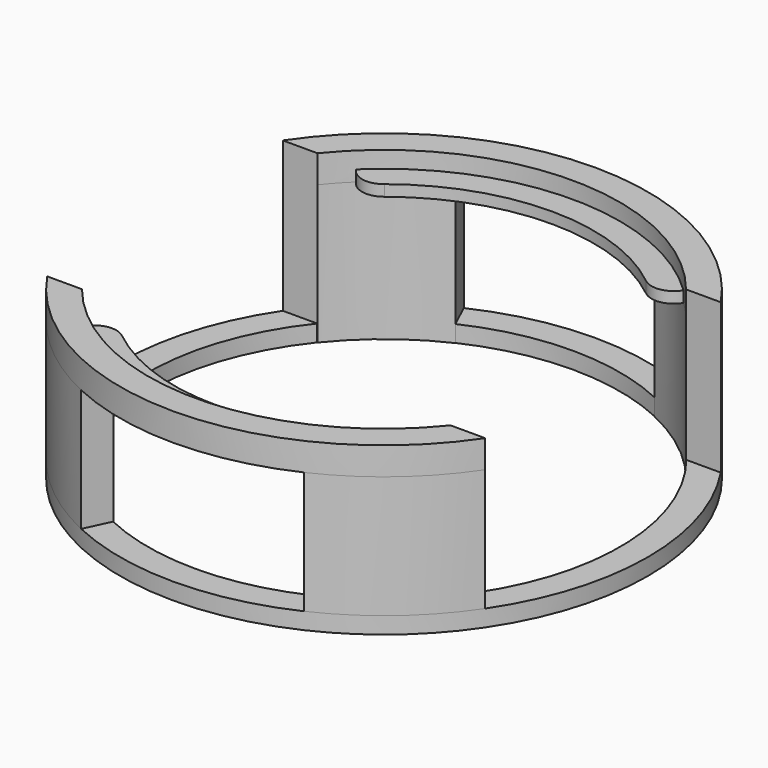
from build123d import *

# Parameters (mm, degrees)
F0_R        = 47.5
F0_R_2      = 42.5
F1_DEPTH    = 3
F3_DEPTH    = 25
F7_DEPTH    = 5
F8_DEPTH    = 2
F9_T1_DEPTH = 43.7405186698


# Not quite as in the source:
# - a fillet or chamfer that OpenCascade refuses, or shapes differently, is made with other operations: its cross-section is extruded or revolved along the edge and cut away or added


with BuildPart() as f1:
    # F0 (on Top) → F1 (new body)
    with BuildSketch(Plane.XY):
        Circle(F0_R)
        Circle(F0_R_2, mode=Mode.SUBTRACT)
    extrude(amount=F1_DEPTH)

    # F2 (on Top) → F3 (join)
    with BuildSketch(Plane.XY):
        with BuildLine():
            Line((-17.9424604553, 38.4777306174), (-20.0743674327, 43.0496198842))
            ThreePointArc((-20.0743674327, 43.0496198842), (-30.8770370262, 36.0951324209), (-39.4208066889, 26.5))
            Line((-39.4208066889, 26.5), (-33.1695287976, 26.5))
            ThreePointArc((-33.1695287976, 26.5), (-26.2483403101, 33.3690316255), (-17.9424604553, 38.4777306174))
        make_face()
        with BuildLine():
            Line((-20.0743674327, -43.0496198842), (-17.9424604553, -38.4777306174))
            ThreePointArc((-17.9424604553, -38.4777306174), (-26.2483403101, -33.3690316255), (-33.1695287976, -26.5))
            Line((-33.1695287976, -26.5), (-39.4208066889, -26.5))
            ThreePointArc((-39.4208066889, -26.5), (-30.8770370262, -36.0951324209), (-20.0743674327, -43.0496198842))
        make_face()
        with BuildLine():
            Line((20.0743674327, 43.0496198842), (17.9424604553, 38.4777306174))
            ThreePointArc((17.9424604553, 38.4777306174), (26.2483403101, 33.3690316255), (33.1695287976, 26.5))
            Line((33.1695287976, 26.5), (39.4208066889, 26.5))
            ThreePointArc((39.4208066889, 26.5), (30.8770370262, 36.0951324209), (20.0743674327, 43.0496198842))
        make_face()
        with BuildLine():
            ThreePointArc((33.1695287976, -26.5), (26.2483403101, -33.3690316255), (17.9424604553, -38.4777306174))
            Line((17.9424604553, -38.4777306174), (20.0743674327, -43.0496198842))
            ThreePointArc((20.0743674327, -43.0496198842), (30.8770370262, -36.0951324209), (39.4208066889, -26.5))
            Line((39.4208066889, -26.5), (33.1695287976, -26.5))
        make_face()
    extrude(amount=F3_DEPTH)

    # F4 (on face) → F7 (join)
    with BuildSketch(Plane.XY.offset(25)):
        with BuildLine():
            ThreePointArc((39.4208066889, 26.5), (0, 47.5), (-39.4208066889, 26.5))
            Line((-39.4208066889, 26.5), (-33.1695287976, 26.5))
            ThreePointArc((-33.1695287976, 26.5), (0, 42.455478335), (33.1695287976, 26.5))
            Line((33.1695287976, 26.5), (39.4208066889, 26.5))
        make_face()
        with BuildLine():
            Line((-33.1695287976, -26.5), (-39.4208066889, -26.5))
            ThreePointArc((-39.4208066889, -26.5), (0, -47.5), (39.4208066889, -26.5))
            Line((39.4208066889, -26.5), (33.1695287976, -26.5))
            ThreePointArc((33.1695287976, -26.5), (0, -42.455478335), (-33.1695287976, -26.5))
        make_face()
    extrude(amount=F7_DEPTH)

    # F6 (on offset) → F8 (join)
    with BuildSketch(Plane.XY.offset(25)):
        with BuildLine():
            ThreePointArc((-29.4712756106, -30.6217882215), (0, -42.5), (29.4712756106, -30.6217882215))
            Line((29.4712756106, -30.6217882215), (29.4712756106, -23.6217882215))
            ThreePointArc((29.4712756106, -23.6217882215), (0, -37.7696301928), (-29.4712756106, -23.6217882215))
            Line((-29.4712756106, -23.6217882215), (-29.4712756106, -30.6217882215))
        make_face()
        with BuildLine():
            Line((29.4712756106, 23.6217882215), (29.4712756106, 30.6217882215))
            ThreePointArc((29.4712756106, 30.6217882215), (0, 42.5), (-29.4712756106, 30.6217882215))
            Line((-29.4712756106, 30.6217882215), (-29.4712756106, 23.6217882215))
            ThreePointArc((-29.4712756106, 23.6217882215), (0, 37.7696301928), (29.4712756106, 23.6217882215))
        make_face()
    extrude(amount=F8_DEPTH)

    # F9: fillet of radius 4 on 4 edges, made by hand

    # F9_s2 → F9_t1 (cut)
    with BuildSketch(Plane.XY.offset(4.1297406651)):
        with BuildLine():
            ThreePointArc((-29.4712756106, -30.5599665337), (-26.7517914385, -28.7057144703), (-23.5623277872, -29.5188359213))
            ThreePointArc((-23.5623277872, -29.5188359213), (-26.6802279831, -26.7340681466), (-29.4712756106, -23.6217882215))
            Line((-29.4712756106, -23.6217882215), (-29.4712756106, -30.5599665337))
        make_face()
        with BuildLine():
            ThreePointArc((23.5623277872, -29.5188359213), (26.7517914385, -28.7057144703), (29.4712756106, -30.5599665337))
            Line((29.4712756106, -30.5599665337), (29.4712756106, -23.6217882215))
            ThreePointArc((29.4712756106, -23.6217882215), (26.6802279831, -26.7340681466), (23.5623277872, -29.5188359213))
        make_face()
        with BuildLine():
            ThreePointArc((29.4712756106, 30.5599665337), (26.7517914385, 28.7057144703), (23.5623277872, 29.5188359213))
            ThreePointArc((23.5623277872, 29.5188359213), (26.6802279831, 26.7340681466), (29.4712756106, 23.6217882215))
            Line((29.4712756106, 23.6217882215), (29.4712756106, 30.5599665337))
        make_face()
        with BuildLine():
            ThreePointArc((-23.5623277872, 29.5188359213), (-26.7517914385, 28.7057144703), (-29.4712756106, 30.5599665337))
            Line((-29.4712756106, 30.5599665337), (-29.4712756106, 23.6217882215))
            ThreePointArc((-29.4712756106, 23.6217882215), (-26.6802279831, 26.7340681466), (-23.5623277872, 29.5188359213))
        make_face()
    extrude(amount=F9_T1_DEPTH, mode=Mode.SUBTRACT)


solid = f1.part
